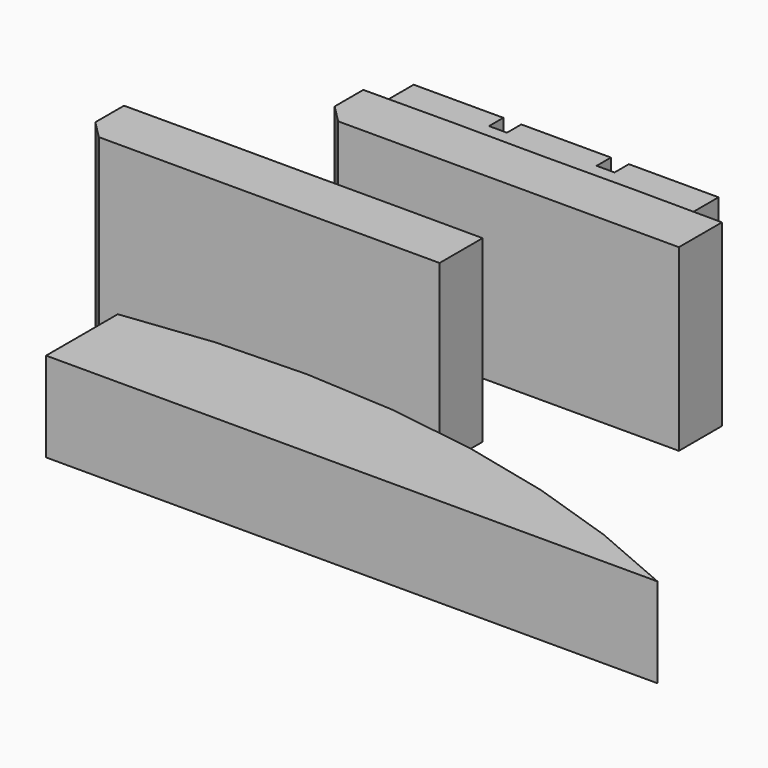
from build123d import *

# Parameters (mm, degrees)
F1_DEPTH  = 0.2
F3_DEPTH  = 0.2
F5_DEPTH  = 5
F7_DEPTH  = 10
F9_DEPTH  = 10
F11_DEPTH = 5


# Not quite as in the source:
# - a feature names something its author has since deleted; it is built from what else it names


with BuildPart() as f1:
    # F0 (on Top) → F1 (new body)
    with BuildSketch(Plane.XY):
        with BuildLine():
            ThreePointArc((-63.7017709232, 41.993062175), (-63.560349567, 42.0516408187), (-63.5017709232, 42.193062175))
            ThreePointArc((-63.5017709232, 42.193062175), (-63.560349567, 42.3344835312), (-63.7017709232, 42.393062175))
            ThreePointArc((-63.7017709232, 42.393062175), (-63.9017709232, 42.193062175), (-63.7017709232, 41.993062175))
        make_face()
        with BuildLine():
            ThreePointArc((-63.7017709232, 42.393062175), (-63.560349567, 42.3344835312), (-63.5017709232, 42.193062175))
            ThreePointArc((-63.5017709232, 42.193062175), (-63.560349567, 42.0516408187), (-63.7017709232, 41.993062175))
            Line((-63.7017709232, 41.993062175), (-61.7017709232, 41.993062175))
            ThreePointArc((-61.7017709232, 41.993062175), (-61.9017709232, 42.193062175), (-61.7017709232, 42.393062175))
            Line((-61.7017709232, 42.393062175), (-63.7017709232, 42.393062175))
        make_face()
        with BuildLine():
            ThreePointArc((-61.5017709232, 42.193062175), (-61.560349567, 42.3344835312), (-61.7017709232, 42.393062175))
            ThreePointArc((-61.7017709232, 42.393062175), (-61.9017709232, 42.193062175), (-61.7017709232, 41.993062175))
            ThreePointArc((-61.7017709232, 41.993062175), (-61.560349567, 42.0516408187), (-61.5017709232, 42.193062175))
        make_face()
    extrude(amount=-F1_DEPTH)


with BuildPart() as f3:
    # F2 (on Top) → F3 (new body)
    with BuildSketch(Plane.XY):
        with BuildLine():
            ThreePointArc((-60.6987384856, 41.9908721328), (-60.5573171293, 42.0494507765), (-60.4987384856, 42.1908721328))
            ThreePointArc((-60.4987384856, 42.1908721328), (-60.5573171293, 42.332293489), (-60.6987384856, 42.3908721328))
            ThreePointArc((-60.6987384856, 42.3908721328), (-60.8987384856, 42.1908721328), (-60.6987384856, 41.9908721328))
        make_face()
        with BuildLine():
            ThreePointArc((-60.6987384856, 41.9908721328), (-60.8987384856, 42.1908721328), (-60.6987384856, 42.3908721328))
            Line((-60.6987384856, 42.3908721328), (-61.6987384856, 42.3908721328))
            ThreePointArc((-61.6987384856, 42.3908721328), (-61.5573171293, 42.332293489), (-61.4987384856, 42.1908721328))
            ThreePointArc((-61.4987384856, 42.1908721328), (-61.5573171293, 42.0494507765), (-61.6987384856, 41.9908721328))
            Line((-61.6987384856, 41.9908721328), (-60.6987384856, 41.9908721328))
        make_face()
        with BuildLine():
            ThreePointArc((-61.4987384856, 42.1908721328), (-61.5573171293, 42.332293489), (-61.6987384856, 42.3908721328))
            ThreePointArc((-61.6987384856, 42.3908721328), (-61.8987384856, 42.1908721328), (-61.6987384856, 41.9908721328))
            ThreePointArc((-61.6987384856, 41.9908721328), (-61.5573171293, 42.0494507765), (-61.4987384856, 42.1908721328))
        make_face()
    extrude(amount=-F3_DEPTH)


with BuildPart() as f5:
    # F4 (on Top) → F5 (new body)
    with BuildSketch(Plane.XY):
        Polygon((-61.6742311418, 37.0802673395), (-66.6742311418, 37.0802673395), (-66.6742311418, 34.0802673395), (-49.6742311418, 34.0802673395), (-49.6742311418, 37.0802673395), (-54.6742311418, 37.0802673395), (-54.6742311418, 36.0802673395), (-55.6742311418, 36.0802673395), (-55.6742311418, 37.0802673395), (-60.6742311418, 37.0802673395), (-60.6742311418, 36.0802673395), (-61.6742311418, 36.0802673395), align=None)
    extrude(amount=F5_DEPTH)


with BuildPart() as f7:
    # F6 (on Top) → F7 (new body)
    with BuildSketch(Plane.XY):
        Polygon((-57.0816621606, 27.8524017553), (-62.0815936218, 27.8262219362), (-62.0815936218, 25.8262219362), (-61.0815936218, 24.8262219362), (-42.0818677769, 24.8262219362), (-42.0818677769, 27.8262219362), (-47.0817992381, 27.8524017553), (-52.0817306994, 27.8262219362), align=None)
    extrude(amount=F7_DEPTH)


with BuildPart() as f9:
    # F8 (on Top) → F9 (new body)
    with BuildSketch(Plane.XY):
        Polygon((-64.2891405681, 20.1605834368), (-69.2891329527, 20.151856795), (-69.2891329527, 18.151856795), (-68.2891329527, 17.151856795), (-49.2891634144, 17.151856795), (-49.2891634144, 20.151856795), (-54.289155799, 20.1605834368), (-59.2891481836, 20.151856795), align=None)
    extrude(amount=F9_DEPTH)


with BuildPart() as f11:
    # F10 (on Top) → F11 (new body)
    with BuildSketch(Plane.XY):
        Polygon((-63.2143030609, 7.1265595207), (-29.1095899709, 7.1265595207), (-33.7004206177, 9.1075375551), (-38.4464353798, 10.6808601151), (-43.3115142192, 11.834553266), (-48.2586309483, 12.5598367065), (-53.2501350215, 12.8511905915), (-58.2480380791, 12.7063975421), (-63.2143030609, 12.1265595207), align=None)
    extrude(amount=F11_DEPTH)


solid = Compound([f1.part, f3.part, f5.part, f7.part, f9.part, f11.part])
